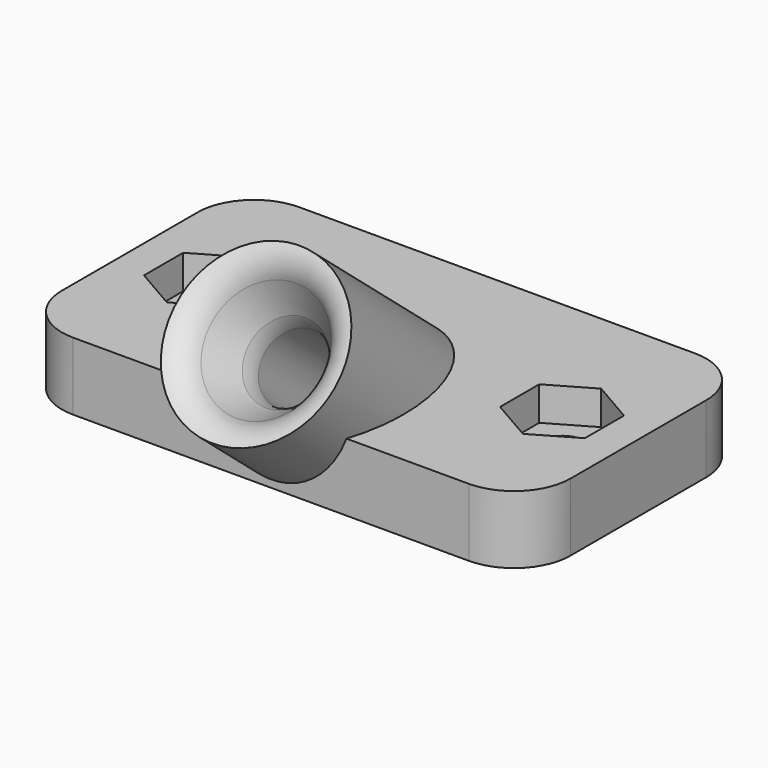
from build123d import *

# Parameters (mm, degrees)
F0_W           = 45
F0_H           = 25
F1_DEPTH       = 6
F2_R           = 5
F5_DEPTH       = 25
F6_R           = 2.1
F7_DEPTH       = 25
F9_R           = 7.5
F10_DEPTH      = 5
F10_DEPTH_BACK = 25
F11_W          = 49.2877000943
F11_H          = 30.2235903218
F12_DEPTH      = 25
F13_W          = 37.6632460393
F13_H          = 10.6945014559
F14_DEPTH      = 25
F15_R          = 3
F16_DEPTH      = 25
F16_DEPTH_BACK = 25
F18_R          = 3


# Not quite as in the source:
# - a fillet or chamfer that OpenCascade refuses, or shapes differently, is made with other operations: its cross-section is extruded or revolved along the edge and cut away or added


with BuildPart() as f1:
    # F0 (on Top) → F1 (new body)
    with BuildSketch(Plane.XY):
        with Locations((22.5, 12.5)):
            Rectangle(F0_W, F0_H)
    extrude(amount=F1_DEPTH)

    # F2
    f2_edges = [f1.edges().sort_by_distance(p)[0] for p in [
        (45, 25, 3),
        (45, 0, 3),
        (0, 25, 3),
        (0, 0, 3),
    ]]
    fillet(f2_edges, radius=F2_R)

    # F4 (on offset) → F5 (cut)
    with BuildSketch(Plane.XY.offset(3)):
        Polygon((3, 14.6650635095), (3, 10.3349364905), (6.75, 8.1698729811), (10.5, 10.3349364905), (10.5, 14.6650635095), (6.75, 16.8301270189), align=None)
        Polygon((42, 10.3349364905), (42, 14.6650635095), (38.25, 16.8301270189), (34.5, 14.6650635095), (34.5, 10.3349364905), (38.25, 8.1698729811), align=None)
    extrude(amount=F5_DEPTH, mode=Mode.SUBTRACT)

    # F6 (on Top) → F7 (cut)
    with BuildSketch(Plane.XY):
        with Locations((6.75, 12.5)):
            Circle(F6_R)
        with Locations((38.25, 12.5)):
            Circle(F6_R)
    extrude(amount=F7_DEPTH, mode=Mode.SUBTRACT)

    # F9 (on face) → F10 (join, two sides)
    with BuildSketch(Plane(origin=(0, -2.954423259, 2.479055467), x_dir=(1, 0, 0), z_dir=(0, -0.7660444431, 0.6427876097))) as f10_sk:
        with Locations((22.5, 8)):
            Circle(F9_R)
    extrude(amount=F10_DEPTH)
    extrude(f10_sk.sketch, amount=-F10_DEPTH_BACK)

    # F11 (on Top) → F12 (cut)
    with BuildSketch(Plane.XY):
        with Locations((22.6797270589, 13.7661970221)):
            Rectangle(F11_W, F11_H)
    extrude(amount=-F12_DEPTH, mode=Mode.SUBTRACT)

    # F13 (on face) → F14 (cut)
    with BuildSketch(Plane(origin=(0, 25, 0), x_dir=(-1, 0, 0), z_dir=(0, 1, 0))):
        with Locations((-22.6992729586, 2.3689556401)):
            Rectangle(F13_W, F13_H)
    extrude(amount=F14_DEPTH, mode=Mode.SUBTRACT)

    # F15 (on face) → F16 (cut, two sides)
    with BuildSketch(Plane(origin=(0, -2.954423259, 2.479055467), x_dir=(1, 0, 0), z_dir=(0, -0.7660444431, 0.6427876097))) as f16_sk:
        with Locations((22.5, 8)):
            Circle(F15_R)
    extrude(amount=F16_DEPTH, mode=Mode.SUBTRACT)
    extrude(f16_sk.sketch, amount=-F16_DEPTH_BACK, mode=Mode.SUBTRACT)

    # F17: chamfer of 3 x 5 on 1 edges, made by hand

    # F17_s1 → F17_t2 (revolve, cut)
    with BuildSketch(Plane(origin=(0, 5.1423008775, 6.128355545), x_dir=(1, 0, 0), z_dir=(0, 0.6427876097, 0.7660444431))):
        Polygon((28.5, -8.8567256581), (25.5, -3.8567256581), (25.5, -8.8567256581), align=None)
    revolve(axis=Axis((22.5, -1.6423445971, 11.8213490604), (0, 0.7660444431, -0.6427876097)), mode=Mode.SUBTRACT)

    # F18
    f18_edges = [f1.edges().sort_by_distance(p)[0] for p in [
        (19.5, 2.187878, 8.607411),
    ]]
    fillet(f18_edges, radius=F18_R)

    # F19: fillet of radius 3 on 1 edges, made by hand

    # F19_s1 → F19_t2 (revolve, cut)
    with BuildSketch(Plane(origin=(0, 5.1423008775, 6.128355545), x_dir=(1, 0, 0), z_dir=(0, 0.6427876097, 0.7660444431))):
        with BuildLine():
            ThreePointArc((27.6302051352, -7.4070675501), (28.6371938466, -8.4227287465), (30, -8.8567256581))
            Line((30, -8.8567256581), (28.5, -8.8567256581))
            Line((28.5, -8.8567256581), (27.6302051352, -7.4070675501))
        make_face()
    revolve(axis=Axis((22.5, -1.6423445971, 11.8213490604), (0, 0.7660444431, -0.6427876097)), mode=Mode.SUBTRACT)


solid = f1.part
